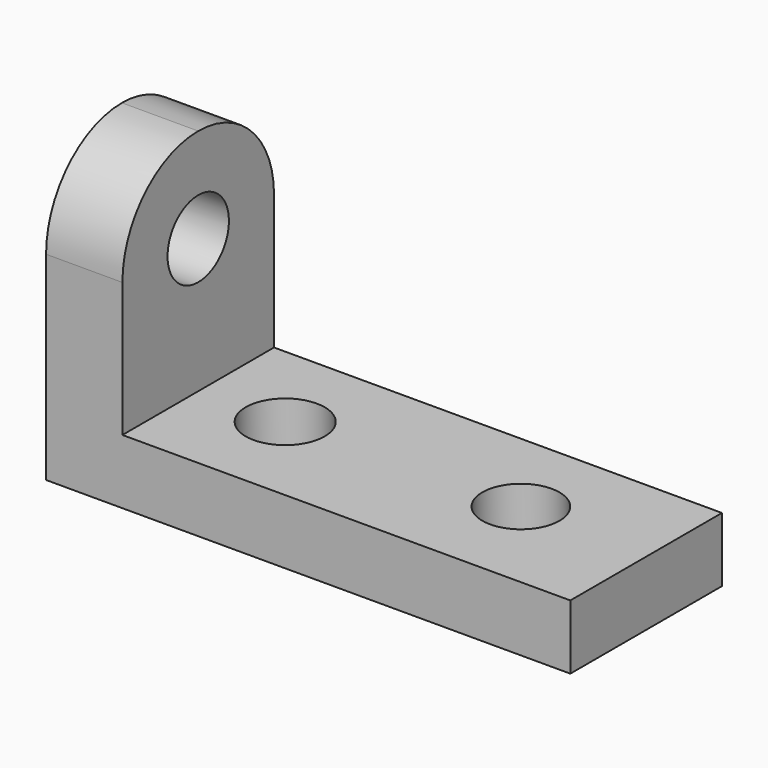
from build123d import *

# Parameters (mm, degrees)
F1_DEPTH = 50
F2_R     = 24.99999
F3_R     = 10.4273095681
F3_R_2   = 10.1761827098
F4_DEPTH = 25
F5_R     = 10.1221707253
F6_DEPTH = 25


# Not quite as in the source:
# - a fillet or chamfer is up to 0.001 mm smaller than in the source, because OpenCascade refuses the exact size


with BuildPart() as f1:
    # F0 (on Front) → F1 (new body)
    with BuildSketch(Plane.XZ):
        Polygon((-87.5170975924, 9.8484745249), (-87.5170975924, -67.5976250101), (50.8091747761, -67.5976250101), (50.8091747761, -50.5853332579), (-67.3725008965, -50.5853332579), (-67.3725008965, 9.8484745249), align=None)
    extrude(amount=F1_DEPTH)

    # F2 (radius 25 in the source; OpenCascade refuses exactly that, so slightly less here)
    f2_edges = [f1.edges().sort_by_distance(p)[0] for p in [
        (-77.444799, -50, 9.848475),
        (-77.444799, 0, 9.848475),
    ]]
    fillet(f2_edges, radius=F2_R)

    # F3 (on face) → F4 (cut)
    with BuildSketch(Plane.XY.offset(-50.5853332579)):
        with Locations((-44.8602624238, -24.4600903243)):
            Circle(F3_R)
        with Locations((16.6889782995, -23.6502327025)):
            Circle(F3_R_2)
    extrude(amount=-F4_DEPTH, mode=Mode.SUBTRACT)

    # F5 (on face) → F6 (cut)
    with BuildSketch(Plane.YZ.offset(-67.3725008965)):
        with Locations((-25, -15.1515254751)):
            Circle(F5_R)
    extrude(amount=-F6_DEPTH, mode=Mode.SUBTRACT)


solid = f1.part
